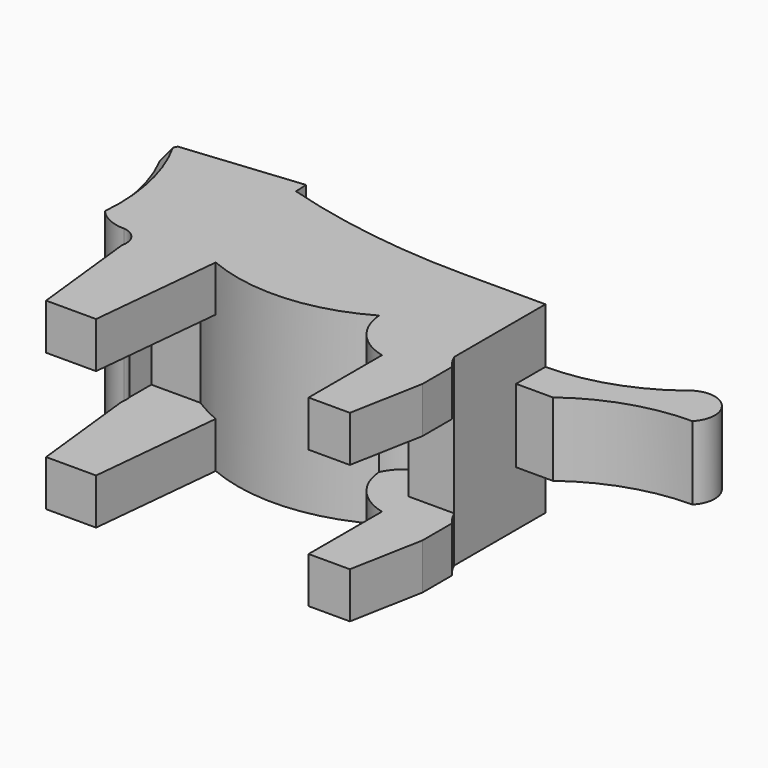
from build123d import *

# Parameters (mm, degrees)
F1_DEPTH     = 25
F2_DEPTH     = 12.5
F4_DEPTH     = 12.5
F5_DEPTH     = 16.25
F7_DEPTH     = 24.3842223705
F6_W         = 10
F6_H         = 10
F8_DEPTH     = 40
F10_DEPTH    = 20
F11_W        = 7.0710678119
F11_H        = 20
F12_ANGLE    = 180
F13_W        = 25
F13_H        = 50
F13_W_2      = 11.2650044263
F14_ANGLE    = 5.7295779513
F15_T1_DEPTH = 52.2024679969
F15_T3_DEPTH = 69.535784442
F15_T6_ANGLE = 45.7032352823
F15_T8_ANGLE = 45.7032352823


# Not quite as in the source:
# - a fillet or chamfer that OpenCascade refuses, or shapes differently, is made with other operations: its cross-section is extruded or revolved along the edge and cut away or added
# - a pattern or mirror of a feature is missing from the dataset's text; its kind, count and spacing are read off the source's solid


with BuildPart() as f1:
    # F0 (on Top) → F1 (new body)
    with BuildSketch(Plane.XY):
        with BuildLine():
            ThreePointArc((8.5724992678, 52.5779476486), (-17.4169661561, 54.4628096646), (-42.8625009954, 60.0779476486))
            Line((-42.8625009954, 60.0779476486), (-79.1275054216, 60.0779476486))
            ThreePointArc((-79.1275054216, 60.0779476486), (-73.2024272044, 46.6744306132), (-71.1757168174, 32.1605315572))
            ThreePointArc((-71.1757168174, 32.1605315572), (-67.4004664777, 26.1656086442), (-60.7126449392, 23.8279476486))
            ThreePointArc((-60.7126449392, 23.8279476486), (-57.8761392565, 22.6699366601), (-56.2426317111, 20.0779476486))
            Line((-56.2426317111, 20.0779476486), (-56.2426317111, 27.5779476486))
            Line((-56.2426317111, 27.5779476486), (-42.8625009954, 27.5779476486))
            ThreePointArc((-42.8625009954, 27.5779476486), (-39.3668172692, 25.5518582213), (-35.7126449392, 23.8279476486))
            ThreePointArc((-35.7126449392, 23.8279476486), (-14.2067307678, 20.1682602333), (6.6882768972, 26.4369372072))
            ThreePointArc((6.6882768972, 26.4369372072), (11.5749679763, 31.8294833583), (18.5724992678, 33.8279476486))
            Line((18.5724992678, 33.8279476486), (18.5724992678, 40.0779476486))
            Line((18.5724992678, 40.0779476486), (18.5724992678, 52.5779476486))
            Line((18.5724992678, 52.5779476486), (8.5724992678, 52.5779476486))
        make_face()
        with BuildLine():
            Line((-56.2426317111, 27.5779476486), (-56.2426317111, 20.0779476486))
            ThreePointArc((-56.2426317111, 20.0779476486), (-56.084348871, 18.8279476486), (-56.2426317111, 17.5779476486))
            Line((-56.2426317111, 17.5779476486), (-52.8975990321, -12.4220523514))
            Line((-52.8975990321, -12.4220523514), (-39.2875729673, -12.4220523514))
            Line((-39.2875729673, -12.4220523514), (-35.7126449392, 23.8279476486))
            ThreePointArc((-35.7126449392, 23.8279476486), (-39.3668172692, 25.5518582213), (-42.8625009954, 27.5779476486))
            Line((-42.8625009954, 27.5779476486), (-56.2426317111, 27.5779476486))
        make_face()
        with BuildLine():
            ThreePointArc((29.8224992678, 27.5779476486), (25.0072681059, 32.1605315572), (18.5724992678, 33.8279476486))
            ThreePointArc((18.5724992678, 33.8279476486), (11.5749679763, 31.8294833583), (6.6882768972, 26.4369372072))
            ThreePointArc((6.6882768972, 26.4369372072), (10.35454594, 17.5558849939), (18.5724992678, 12.5779476486))
            Line((18.5724992678, 12.5779476486), (18.5724992678, -12.4220523514))
            Line((18.5724992678, -12.4220523514), (29.8224992678, -12.4220523514))
            Line((29.8224992678, -12.4220523514), (33.5724992678, 7.5779476486))
            Line((33.5724992678, 7.5779476486), (33.5724992678, 17.5779476486))
            ThreePointArc((33.5724992678, 17.5779476486), (30.7908263589, 22.2379453078), (29.8224992678, 27.5779476486))
        make_face()
    extrude(amount=F1_DEPTH)

    # F0 (on Top) → F2 (cut)
    with BuildSketch(Plane.XY):
        with BuildLine():
            ThreePointArc((29.8224992678, 27.5779476486), (25.0072681059, 32.1605315572), (18.5724992678, 33.8279476486))
            ThreePointArc((18.5724992678, 33.8279476486), (11.5749679763, 31.8294833583), (6.6882768972, 26.4369372072))
            ThreePointArc((6.6882768972, 26.4369372072), (10.35454594, 17.5558849939), (18.5724992678, 12.5779476486))
            Line((18.5724992678, 12.5779476486), (18.5724992678, -12.4220523514))
            Line((18.5724992678, -12.4220523514), (29.8224992678, -12.4220523514))
            Line((29.8224992678, -12.4220523514), (33.5724992678, 7.5779476486))
            Line((33.5724992678, 7.5779476486), (33.5724992678, 17.5779476486))
            ThreePointArc((33.5724992678, 17.5779476486), (30.7908263589, 22.2379453078), (29.8224992678, 27.5779476486))
        make_face()
        with BuildLine():
            Line((-56.2426317111, 27.5779476486), (-56.2426317111, 20.0779476486))
            ThreePointArc((-56.2426317111, 20.0779476486), (-56.084348871, 18.8279476486), (-56.2426317111, 17.5779476486))
            Line((-56.2426317111, 17.5779476486), (-52.8975990321, -12.4220523514))
            Line((-52.8975990321, -12.4220523514), (-39.2875729673, -12.4220523514))
            Line((-39.2875729673, -12.4220523514), (-35.7126449392, 23.8279476486))
            ThreePointArc((-35.7126449392, 23.8279476486), (-39.3668172692, 25.5518582213), (-42.8625009954, 27.5779476486))
            Line((-42.8625009954, 27.5779476486), (-56.2426317111, 27.5779476486))
        make_face()
    extrude(amount=F2_DEPTH, mode=Mode.SUBTRACT)

    # F3: F1 across plane


with BuildPart() as f1_1:
    add(f1.part)
    add(f1.part.mirror(Plane.XY))

    # F4 (add): a face of the model
    f4_faces = [f1_1.faces().sort_by_distance(p)[0] for p in [
        (18.5724992678, 43.2029476486, 0),
    ]]
    extrude(f4_faces, amount=F4_DEPTH)

    # F5 (add, through all): a face of the model
    f5_faces = [f1_1.faces().sort_by_distance(p)[0] for p in [
        (24.8224992678, 33.8279476486, 0),
    ]]
    extrude(f5_faces, amount=F5_DEPTH)

    # F6 (on face) → F7 (cut, through all)
    with BuildSketch(Plane.YZ.offset(31.0724992678)):
        Polygon((21.5398740044, 0), (21.5398740044, 12.5), (17.5779476486, 12.5), (17.5779476486, -12.5), (21.5398740044, -12.5), align=None)
    extrude(amount=-F7_DEPTH, mode=Mode.SUBTRACT)

    # F6 (on face) → F8 (join)
    with BuildSketch(Plane.YZ.offset(31.0724992678)):
        Polygon((62.5779476486, 10), (52.5779476486, 10), (52.5779476486, 0), (52.5779476486, -10), (62.5779476486, -10), align=None)
        with Locations((47.5779476486, 5)):
            Rectangle(F6_W, F6_H)
    f8 = extrude(amount=F8_DEPTH)

    # F8_copies: F8 across plane
    add(f8.mirror(Plane(origin=(0, 0, 0), x_dir=(-1, 0, 0), z_dir=(0, 0, -1))))

    # F9 (on face) → F10 (cut, through all)
    with BuildSketch(Plane.XY.offset(10)):
        with BuildLine():
            ThreePointArc((31.0724992678, 52.5779476486), (46.8838875686, 55.1437827461), (61.0724992678, 62.5779476486))
            Line((61.0724992678, 62.5779476486), (51.0724992678, 62.5779476486))
            Line((51.0724992678, 62.5779476486), (31.0724992678, 62.5779476486))
            Line((31.0724992678, 62.5779476486), (31.0724992678, 52.5779476486))
        make_face()
        Polygon((71.0724992678, 52.5779476486), (71.0724992678, 62.5779476486), (61.0724992678, 62.5779476486), align=None)
        with BuildLine():
            Line((71.0724992678, 42.5779476486), (71.0724992678, 52.5779476486))
            ThreePointArc((71.0724992678, 52.5779476486), (55.2611109669, 50.0121125511), (41.0724992678, 42.5779476486))
            Line((41.0724992678, 42.5779476486), (51.0724992678, 42.5779476486))
            Line((51.0724992678, 42.5779476486), (71.0724992678, 42.5779476486))
        make_face()
    extrude(amount=-F10_DEPTH, mode=Mode.SUBTRACT)

    # F11 (on face) → F12 (revolve)
    with BuildSketch(Plane(origin=(61.8252234582, 61.8252234582, 0), x_dir=(-0.7071067812, 0.7071067812, 0), z_dir=(0.7071067812, 0.7071067812, 0))):
        with Locations((-2.4710211471, 0)):
            Rectangle(F11_W, F11_H)
    revolve(axis=Axis((66.0724992678, 57.5779476486, 0), (0, 0, -1)), revolution_arc=F12_ANGLE)

    # F13 (on face) → F14 (revolve)
    with BuildSketch(Plane(origin=(0, 60.0779476486, 0), x_dir=(-1, 0, 0), z_dir=(0, 1, 0))):
        with Locations((55.3625009954, 0)):
            Rectangle(F13_W, F13_H)
        with Locations((73.4950032085, 0)):
            Rectangle(F13_W_2, F13_H)
    revolve(axis=Axis((-79.1275054216, 60.0779476486, 0), (0, 0, 1)), revolution_arc=F14_ANGLE)

    # F15: chamfer of 2.5 on 4 edges, made by hand

    # F15_s2 → F15_t1 (cut)
    with BuildSketch(Plane.XY.offset(-26.1012339984)):
        with BuildLine():
            Line((-71.1765205144, 32.4523590493), (-71.0941336441, 31.829473599))
            ThreePointArc((-71.0941336441, 31.829473599), (-71.1242415299, 31.9464717064), (-71.1757168174, 32.1605315572))
            ThreePointArc((-71.1757168174, 32.1605315572), (-71.1760775289, 32.3560379433), (-71.1765205144, 32.4523590493))
        make_face()
    extrude(amount=F15_T1_DEPTH, mode=Mode.SUBTRACT)

    # F15_s4 → F15_t3 (cut)
    with BuildSketch(Plane.XY.offset(-34.767892221)):
        with BuildLine():
            Line((-77.2597253727, 56.8116607658), (-75.2963846316, 60.4623418968))
            Line((-75.2963846316, 60.4623418968), (-79.1275054216, 60.0779476486))
            ThreePointArc((-79.1275054216, 60.0779476486), (-78.1514580859, 58.4383743549), (-77.2597253727, 56.8116607658))
        make_face()
    extrude(amount=F15_T3_DEPTH, mode=Mode.SUBTRACT)

    # F15_s5 → F15_t6 (revolve, cut)
    with BuildSketch(Plane(origin=(-64.3425340859, 80.1682893814, 0), x_dir=(0, 0, 1), z_dir=(-0.6259274923, 0.7798812566, 0))):
        Polygon((22.5, -23.7159805894), (25, -21.2159805894), (25, -23.7159805894), align=None)
    revolve(axis=Axis((-124.1583289793, 32.1605315572, 25), (0, 0, -1)), revolution_arc=F15_T6_ANGLE, mode=Mode.SUBTRACT)

    # F15_s7 → F15_t8 (revolve, cut)
    with BuildSketch(Plane(origin=(-64.3425340859, 80.1682893814, 0), x_dir=(0, 0, 1), z_dir=(-0.6259274923, 0.7798812566, 0))):
        Polygon((-25, -21.2159805894), (-22.5, -23.7159805894), (-25, -23.7159805894), align=None)
    revolve(axis=Axis((-124.1583289793, 32.1605315572, -25), (0, 0, -1)), revolution_arc=F15_T8_ANGLE, mode=Mode.SUBTRACT)


solid = f1_1.part
